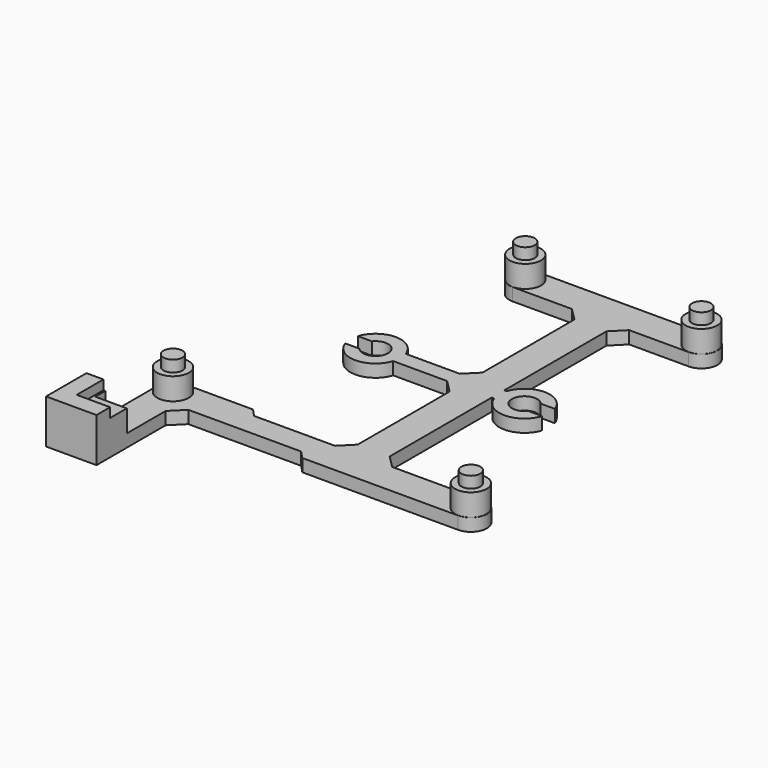
from build123d import *

# Parameters (mm, degrees)
F1_DEPTH  = 2
F3_DEPTH  = 7
F4_R      = 2.5
F4_W      = 5
F4_H      = 3
F5_DEPTH  = 5.5
F6_R      = 1.5
F7_DEPTH  = 1.8
F9_DEPTH  = 1.5
F10_SIZE  = 2
F12_DEPTH = 2
F13_SIZE  = 2


# Not quite as in the source:
# - a feature names something its author has since deleted; it is built from what else it names


with BuildPart() as f1:
    # F0 (on Top) → F1 (new body)
    with BuildSketch(Plane.XY):
        with BuildLine():
            Line((2.46, -15.24), (2.46, -2.54))
            Line((2.46, -2.54), (22.3642048012, -2.54))
            Line((22.3642048012, -2.54), (23.5517361372, -3.81))
            Line((23.5517361372, -3.81), (48.26, -3.81))
            ThreePointArc((48.26, -3.81), (50.8, -1.27), (48.26, 1.27))
            Line((48.26, 1.27), (31.75, 1.27))
            Line((31.75, 1.27), (31.75, 48.26))
            Line((31.75, 48.26), (43.18, 48.26))
            ThreePointArc((43.18, 48.26), (45.72, 50.8), (43.18, 53.34))
            Line((43.18, 53.34), (15.24, 53.34))
            ThreePointArc((15.24, 53.34), (12.7, 50.8), (15.24, 48.26))
            Line((15.24, 48.26), (26.67, 48.26))
            Line((26.67, 48.26), (26.67, 1.27))
            Line((26.67, 1.27), (11.8467498474, 1.27))
            Line((11.8467498474, 1.27), (10.6592185114, 2.54))
            Line((10.6592185114, 2.54), (0, 2.54))
            ThreePointArc((0, 2.54), (-1.7960512242, 1.7960512242), (-2.54, 0))
            Line((-2.54, 0), (-2.54, -15.24))
            Line((-2.54, -15.24), (2.46, -15.24))
        make_face()
    extrude(amount=F1_DEPTH)

    # F2 (on Top) → F3 (join)
    with BuildSketch(Plane.XY):
        Polygon((2.46, -18.24), (2.46, -15.24), (-2.54, -15.24), (-2.54, -10.24), (-5.54, -10.24), (-5.54, -18.24), align=None)
    extrude(amount=F3_DEPTH)

    # F4 (on Top) → F5 (join)
    with BuildSketch(Plane.XY):
        Circle(F4_R)
        with Locations((48.26, -1.27)):
            Circle(F4_R)
        with Locations((15.24, 50.8)):
            Circle(F4_R)
        with Locations((43.18, 50.8)):
            Circle(F4_R)
        with Locations((-0.04, -13.74)):
            Rectangle(F4_W, F4_H)
    extrude(amount=F5_DEPTH)

    # F6 (on face) → F7 (join)
    with BuildSketch(Plane.XY.offset(5.5)):
        Circle(F6_R)
        with Locations((48.26, -1.27)):
            Circle(F6_R)
        with Locations((15.24, 50.8)):
            Circle(F6_R)
        with Locations((43.18, 50.8)):
            Circle(F6_R)
    extrude(amount=F7_DEPTH)

    # F8 (on face) → F9 (cut)
    with BuildSketch(Plane.XY.offset(7)):
        Polygon((2.46, -15.24), (-2.54, -15.24), (-2.54, -10.24), (-2.84, -10.24), (-2.84, -15.54), (2.46, -15.54), align=None)
    extrude(amount=-F9_DEPTH, mode=Mode.SUBTRACT)

    # F10
    f10_edges = [f1.edges().sort_by_distance(p)[0] for p in [
        (31.75, 48.26, 1),
        (26.67, 48.26, 1),
        (26.67, 1.27, 1),
        (31.75, 1.27, 1),
        (2.46, -2.54, 1),
    ]]
    chamfer(f10_edges, length=F10_SIZE)

    # F11 (on Top) → F12 (join)
    with BuildSketch(Plane.XY):
        with BuildLine():
            ThreePointArc((37.5112494996, 23.515), (33.95, 24.765), (37.5112494996, 26.015))
            Line((37.5112494996, 26.015), (39.7496710384, 26.015))
            ThreePointArc((39.7496710384, 26.015), (35.95, 28.765), (32.1503289616, 26.015))
            ThreePointArc((32.1503289616, 26.015), (31.95, 24.765), (32.1503289616, 23.515))
            ThreePointArc((32.1503289616, 23.515), (35.95, 20.765), (39.7496710384, 23.515))
            Line((39.7496710384, 23.515), (37.5112494996, 23.515))
        make_face()
        with BuildLine():
            ThreePointArc((32.1503289616, 23.515), (31.95, 24.765), (32.1503289616, 26.015))
            Line((32.1503289616, 26.015), (31.75, 26.015))
            Line((31.75, 26.015), (31.75, 23.515))
            Line((31.75, 23.515), (32.1503289616, 23.515))
        make_face()
        with BuildLine():
            ThreePointArc((16.1096710384, 26.015), (12.31, 28.765), (8.5103289616, 26.015))
            Line((8.5103289616, 26.015), (10.7487505004, 26.015))
            ThreePointArc((10.7487505004, 26.015), (14.31, 24.765), (10.7487505004, 23.515))
            Line((10.7487505004, 23.515), (8.5103289616, 23.515))
            ThreePointArc((8.5103289616, 23.515), (12.31, 20.765), (16.1096710384, 23.515))
            ThreePointArc((16.1096710384, 23.515), (16.31, 24.765), (16.1096710384, 26.015))
        make_face()
        with BuildLine():
            Line((26.67, 26.015), (16.1096710384, 26.015))
            ThreePointArc((16.1096710384, 26.015), (16.31, 24.765), (16.1096710384, 23.515))
            Line((16.1096710384, 23.515), (26.67, 23.515))
            Line((26.67, 23.515), (26.67, 26.015))
        make_face()
    extrude(amount=F12_DEPTH)

    # F13
    f13_edges = [f1.edges().sort_by_distance(p)[0] for p in [
        (26.67, 23.515, 1),
        (26.67, 26.015, 1),
    ]]
    chamfer(f13_edges, length=F13_SIZE)


solid = f1.part
